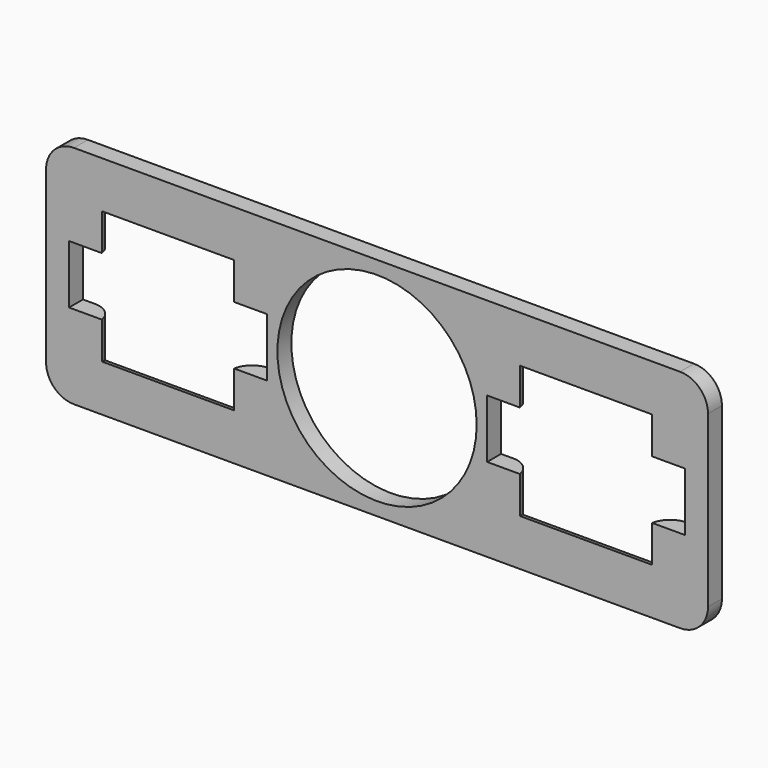
from build123d import *

# Parameters (mm, degrees)
F0_W          = 120.65
F0_H          = 41.148
F0_R          = 18.161
F1_DEPTH      = 3.175
F2_T1_DEPTH   = 24.13
F2_T3_DEPTH   = 16.1227766557
F2_T5_DEPTH   = 24.13
F2_T7_DEPTH   = 16.1227766557
F2_T13_DEPTH  = 16.1227766557
F2_T18_DEPTH  = 33.5217766557
F2_T25_DEPTH  = 33.5217766557
F2_T29_DEPTH  = 16.1227766557
F2_T37_DEPTH  = 33.5217766557
F2_T41_DEPTH  = 16.1227766557
F2_T49_DEPTH  = 16.1227766557
F2_T54_DEPTH  = 33.5217766557
F2_T61_DEPTH  = 33.5217766557
F2_T65_DEPTH  = 16.1227766557
F2_T73_DEPTH  = 16.1227766557
F2_T78_DEPTH  = 33.5217766557
F2_T85_DEPTH  = 33.5217766557
F2_T89_DEPTH  = 16.1227766557
F2_T97_DEPTH  = 16.1227766557
F2_T102_DEPTH = 33.5217766557
F3_R          = 5.08


# Not quite as in the source:
# - a fillet or chamfer that OpenCascade refuses, or shapes differently, is made with other operations: its cross-section is extruded or revolved along the edge and cut away or added
# - a feature names something its author has since deleted; it is built from what else it names


with BuildPart() as f1:
    # F0 (on Front) → F1 (new body)
    with BuildSketch(Plane.XZ):
        Rectangle(F0_W, F0_H)
        Polygon((-26.035, 5.334), (-20.066, 5.334), (-20.066, -5.334), (-26.035, -5.334), (-26.035, -12.065), (-50.165, -12.065), (-50.165, -5.334), (-56.134, -5.334), (-56.134, 5.334), (-50.165, 5.334), (-50.165, 12.065), (-26.035, 12.065), align=None, mode=Mode.SUBTRACT)
        Circle(F0_R, mode=Mode.SUBTRACT)
        Polygon((50.165, 5.334), (56.134, 5.334), (56.134, -5.334), (50.165, -5.334), (50.165, -12.065), (26.035, -12.065), (26.035, -5.334), (20.066, -5.334), (20.066, 5.334), (26.035, 5.334), (26.035, 12.065), (50.165, 12.065), align=None, mode=Mode.SUBTRACT)
    extrude(amount=F1_DEPTH)

    # F2: fillet of radius 3.81 on 12 edges, made by hand

    # F2_s2 → F2_t1 (cut)
    with BuildSketch(Plane.YZ.offset(26.035)):
        with BuildLine():
            ThreePointArc((-3.175, 12.065), (-0.9000644337, 13.3623662374), (0, 15.8217106623))
            Line((0, 15.8217106623), (0, 12.065))
            Line((0, 12.065), (-3.175, 12.065))
        make_face()
        with BuildLine():
            ThreePointArc((-3.175, -12.065), (-0.9000644337, -13.3623662374), (0, -15.8217106623))
            Line((0, -15.8217106623), (0, -12.065))
            Line((0, -12.065), (-3.175, -12.065))
        make_face()
    extrude(amount=F2_T1_DEPTH, mode=Mode.SUBTRACT)

    # F2_s4 → F2_t3 (cut)
    with BuildSketch(Plane.XY.offset(-4.0577766557)):
        with BuildLine():
            ThreePointArc((26.035, -3.175), (24.7376337626, -0.9000644337), (22.2782893377, 0))
            Line((22.2782893377, 0), (26.035, 0))
            Line((26.035, 0), (26.035, -3.175))
        make_face()
        with BuildLine():
            ThreePointArc((50.165, -3.175), (51.4623662374, -0.9000644337), (53.9217106623, 0))
            Line((53.9217106623, 0), (50.165, 0))
            Line((50.165, 0), (50.165, -3.175))
        make_face()
        with BuildLine():
            ThreePointArc((-26.035, -3.175), (-24.7376337626, -0.9000644337), (-22.2782893377, 0))
            Line((-22.2782893377, 0), (-26.035, 0))
            Line((-26.035, 0), (-26.035, -3.175))
        make_face()
        with BuildLine():
            ThreePointArc((-50.165, -3.175), (-51.4623662374, -0.9000644337), (-53.9217106623, 0))
            Line((-53.9217106623, 0), (-50.165, 0))
            Line((-50.165, 0), (-50.165, -3.175))
        make_face()
    extrude(amount=F2_T3_DEPTH, mode=Mode.SUBTRACT)

    # F2_s6 → F2_t5 (cut)
    with BuildSketch(Plane.YZ.offset(-50.165)):
        with BuildLine():
            ThreePointArc((-3.175, 12.065), (-0.9000644337, 13.3623662374), (0, 15.8217106623))
            Line((0, 15.8217106623), (0, 12.065))
            Line((0, 12.065), (-3.175, 12.065))
        make_face()
        with BuildLine():
            ThreePointArc((-3.175, -12.065), (-0.9000644337, -13.3623662374), (0, -15.8217106623))
            Line((0, -15.8217106623), (0, -12.065))
            Line((0, -12.065), (-3.175, -12.065))
        make_face()
    extrude(amount=F2_T5_DEPTH, mode=Mode.SUBTRACT)

    # F2_s8 → F2_t7 (cut)
    with BuildSketch(Plane.XY.offset(-12.065)):
        with BuildLine():
            ThreePointArc((-50.165, -3.175), (-51.4623662374, -0.9000644337), (-53.9217106623, 0))
            Line((-53.9217106623, 0), (-50.165, 0))
            Line((-50.165, 0), (-50.165, -3.175))
        make_face()
        with BuildLine():
            ThreePointArc((-26.035, -3.175), (-24.7376337626, -0.9000644337), (-22.2782893377, 0))
            Line((-22.2782893377, 0), (-26.035, 0))
            Line((-26.035, 0), (-26.035, -3.175))
        make_face()
        with BuildLine():
            ThreePointArc((26.035, -3.175), (24.7376337626, -0.9000644337), (22.2782893377, 0))
            Line((22.2782893377, 0), (26.035, 0))
            Line((26.035, 0), (26.035, -3.175))
        make_face()
        with BuildLine():
            ThreePointArc((50.165, -3.175), (51.4623662374, -0.9000644337), (53.9217106623, 0))
            Line((53.9217106623, 0), (50.165, 0))
            Line((50.165, 0), (50.165, -3.175))
        make_face()
    extrude(amount=F2_T7_DEPTH, mode=Mode.SUBTRACT)


with BuildPart() as f2_tool11:
    # F2_s12 → F2_t13 (new body)
    with BuildSketch(Plane.XY.offset(5.334)):
        with BuildLine():
            ThreePointArc((26.035, -3.175), (24.7376337626, -0.9000644337), (22.2782893377, 0))
            Line((22.2782893377, 0), (26.035, 0))
            Line((26.035, 0), (26.035, -3.175))
        make_face()
    extrude(amount=F2_T13_DEPTH)

    split(bisect_by=Plane.XY.offset(20.574), keep=Keep.BOTTOM)

    split(bisect_by=Plane.XY.offset(12.065), keep=Keep.TOP)


with BuildPart() as f2_tool16:
    # F2_s17 → F2_t18 (new body)
    with BuildSketch(Plane.YZ.offset(16.6432233443)):
        with BuildLine():
            ThreePointArc((-3.175, 12.065), (-0.9000644337, 13.3623662374), (0, 15.8217106623))
            Line((0, 15.8217106623), (0, 12.065))
            Line((0, 12.065), (-3.175, 12.065))
        make_face()
    extrude(amount=F2_T18_DEPTH)

    split(bisect_by=Plane.YZ.offset(26.035), keep=Keep.BOTTOM)


with BuildPart() as f2_tool11_1:
    add(f2_tool11.part)

    # F2_t20: intersect F2_tool16
    add(f2_tool16.part, mode=Mode.INTERSECT)


with BuildPart() as f1_1:
    add(f1.part)

    # F2_t9: cut F2_tool11
    add(f2_tool11_1.part, mode=Mode.SUBTRACT)


with BuildPart() as f2_tool23:
    # F2_s24 → F2_t25 (new body)
    with BuildSketch(Plane.YZ.offset(26.035)):
        with BuildLine():
            ThreePointArc((-3.175, 12.065), (-0.9000644337, 13.3623662374), (0, 15.8217106623))
            Line((0, 15.8217106623), (0, 12.065))
            Line((0, 12.065), (-3.175, 12.065))
        make_face()
    extrude(amount=F2_T25_DEPTH)

    split(bisect_by=Plane.YZ.offset(50.165), keep=Keep.TOP)


with BuildPart() as f2_tool27:
    # F2_s28 → F2_t29 (new body)
    with BuildSketch(Plane.XY.offset(21.4567766557)):
        with BuildLine():
            ThreePointArc((50.165, -3.175), (51.4623662374, -0.9000644337), (53.9217106623, 0))
            Line((53.9217106623, 0), (50.165, 0))
            Line((50.165, 0), (50.165, -3.175))
        make_face()
    extrude(amount=-F2_T29_DEPTH)

    split(bisect_by=Plane.XY.offset(20.574), keep=Keep.BOTTOM)

    split(bisect_by=Plane.XY.offset(12.065), keep=Keep.TOP)


with BuildPart() as f2_tool23_1:
    add(f2_tool23.part)

    # F2_t32: intersect F2_tool27
    add(f2_tool27.part, mode=Mode.INTERSECT)


with BuildPart() as f1_2:
    add(f1_1.part)

    # F2_t21: cut F2_tool23
    add(f2_tool23_1.part, mode=Mode.SUBTRACT)


with BuildPart() as f2_tool35:
    # F2_s36 → F2_t37 (new body)
    with BuildSketch(Plane.YZ.offset(-50.165)):
        with BuildLine():
            ThreePointArc((-3.175, 12.065), (-0.9000644337, 13.3623662374), (0, 15.8217106623))
            Line((0, 15.8217106623), (0, 12.065))
            Line((0, 12.065), (-3.175, 12.065))
        make_face()
    extrude(amount=F2_T37_DEPTH)

    split(bisect_by=Plane.YZ.offset(-26.035), keep=Keep.TOP)


with BuildPart() as f2_tool39:
    # F2_s40 → F2_t41 (new body)
    with BuildSketch(Plane.XY.offset(21.4567766557)):
        with BuildLine():
            ThreePointArc((-26.035, -3.175), (-24.7376337626, -0.9000644337), (-22.2782893377, 0))
            Line((-22.2782893377, 0), (-26.035, 0))
            Line((-26.035, 0), (-26.035, -3.175))
        make_face()
    extrude(amount=-F2_T41_DEPTH)

    split(bisect_by=Plane.XY.offset(20.574), keep=Keep.BOTTOM)

    split(bisect_by=Plane.XY.offset(12.065), keep=Keep.TOP)


with BuildPart() as f2_tool35_1:
    add(f2_tool35.part)

    # F2_t44: intersect F2_tool39
    add(f2_tool39.part, mode=Mode.INTERSECT)


with BuildPart() as f1_3:
    add(f1_2.part)

    # F2_t33: cut F2_tool35
    add(f2_tool35_1.part, mode=Mode.SUBTRACT)


with BuildPart() as f2_tool47:
    # F2_s48 → F2_t49 (new body)
    with BuildSketch(Plane.XY.offset(5.334)):
        with BuildLine():
            ThreePointArc((-50.165, -3.175), (-51.4623662374, -0.9000644337), (-53.9217106623, 0))
            Line((-53.9217106623, 0), (-50.165, 0))
            Line((-50.165, 0), (-50.165, -3.175))
        make_face()
    extrude(amount=F2_T49_DEPTH)

    split(bisect_by=Plane.XY.offset(20.574), keep=Keep.BOTTOM)

    split(bisect_by=Plane.XY.offset(12.065), keep=Keep.TOP)


with BuildPart() as f2_tool52:
    # F2_s53 → F2_t54 (new body)
    with BuildSketch(Plane.YZ.offset(-59.5567766557)):
        with BuildLine():
            ThreePointArc((-3.175, 12.065), (-0.9000644337, 13.3623662374), (0, 15.8217106623))
            Line((0, 15.8217106623), (0, 12.065))
            Line((0, 12.065), (-3.175, 12.065))
        make_face()
    extrude(amount=F2_T54_DEPTH)

    split(bisect_by=Plane.YZ.offset(-50.165), keep=Keep.BOTTOM)


with BuildPart() as f2_tool47_1:
    add(f2_tool47.part)

    # F2_t56: intersect F2_tool52
    add(f2_tool52.part, mode=Mode.INTERSECT)


with BuildPart() as f1_4:
    add(f1_3.part)

    # F2_t45: cut F2_tool47
    add(f2_tool47_1.part, mode=Mode.SUBTRACT)


with BuildPart() as f2_tool59:
    # F2_s60 → F2_t61 (new body)
    with BuildSketch(Plane.YZ.offset(-26.035)):
        with BuildLine():
            ThreePointArc((-3.175, -12.065), (-0.9000644337, -13.3623662374), (0, -15.8217106623))
            Line((0, -15.8217106623), (0, -12.065))
            Line((0, -12.065), (-3.175, -12.065))
        make_face()
    extrude(amount=-F2_T61_DEPTH)

    split(bisect_by=Plane.YZ.offset(-50.165), keep=Keep.BOTTOM)


with BuildPart() as f2_tool63:
    # F2_s64 → F2_t65 (new body)
    with BuildSketch(Plane.XY.offset(-21.4567766557)):
        with BuildLine():
            ThreePointArc((-50.165, -3.175), (-51.4623662374, -0.9000644337), (-53.9217106623, 0))
            Line((-53.9217106623, 0), (-50.165, 0))
            Line((-50.165, 0), (-50.165, -3.175))
        make_face()
    extrude(amount=F2_T65_DEPTH)

    split(bisect_by=Plane.XY.offset(-20.574), keep=Keep.TOP)

    split(bisect_by=Plane.XY.offset(-12.065), keep=Keep.BOTTOM)


with BuildPart() as f2_tool59_1:
    add(f2_tool59.part)

    # F2_t68: intersect F2_tool63
    add(f2_tool63.part, mode=Mode.INTERSECT)


with BuildPart() as f1_5:
    add(f1_4.part)

    # F2_t57: cut F2_tool59
    add(f2_tool59_1.part, mode=Mode.SUBTRACT)


with BuildPart() as f2_tool71:
    # F2_s72 → F2_t73 (new body)
    with BuildSketch(Plane.XY.offset(-5.334)):
        with BuildLine():
            ThreePointArc((-26.035, -3.175), (-24.7376337626, -0.9000644337), (-22.2782893377, 0))
            Line((-22.2782893377, 0), (-26.035, 0))
            Line((-26.035, 0), (-26.035, -3.175))
        make_face()
    extrude(amount=-F2_T73_DEPTH)

    split(bisect_by=Plane.XY.offset(-20.574), keep=Keep.TOP)

    split(bisect_by=Plane.XY.offset(-12.065), keep=Keep.BOTTOM)


with BuildPart() as f2_tool76:
    # F2_s77 → F2_t78 (new body)
    with BuildSketch(Plane.YZ.offset(-16.6432233443)):
        with BuildLine():
            ThreePointArc((-3.175, -12.065), (-0.9000644337, -13.3623662374), (0, -15.8217106623))
            Line((0, -15.8217106623), (0, -12.065))
            Line((0, -12.065), (-3.175, -12.065))
        make_face()
    extrude(amount=-F2_T78_DEPTH)

    split(bisect_by=Plane.YZ.offset(-26.035), keep=Keep.TOP)


with BuildPart() as f2_tool71_1:
    add(f2_tool71.part)

    # F2_t80: intersect F2_tool76
    add(f2_tool76.part, mode=Mode.INTERSECT)


with BuildPart() as f1_6:
    add(f1_5.part)

    # F2_t69: cut F2_tool71
    add(f2_tool71_1.part, mode=Mode.SUBTRACT)


with BuildPart() as f2_tool83:
    # F2_s84 → F2_t85 (new body)
    with BuildSketch(Plane.YZ.offset(50.165)):
        with BuildLine():
            ThreePointArc((-3.175, -12.065), (-0.9000644337, -13.3623662374), (0, -15.8217106623))
            Line((0, -15.8217106623), (0, -12.065))
            Line((0, -12.065), (-3.175, -12.065))
        make_face()
    extrude(amount=-F2_T85_DEPTH)

    split(bisect_by=Plane.YZ.offset(26.035), keep=Keep.BOTTOM)


with BuildPart() as f2_tool87:
    # F2_s88 → F2_t89 (new body)
    with BuildSketch(Plane.XY.offset(-21.4567766557)):
        with BuildLine():
            ThreePointArc((26.035, -3.175), (24.7376337626, -0.9000644337), (22.2782893377, 0))
            Line((22.2782893377, 0), (26.035, 0))
            Line((26.035, 0), (26.035, -3.175))
        make_face()
    extrude(amount=F2_T89_DEPTH)

    split(bisect_by=Plane.XY.offset(-20.574), keep=Keep.TOP)

    split(bisect_by=Plane.XY.offset(-12.065), keep=Keep.BOTTOM)


with BuildPart() as f2_tool83_1:
    add(f2_tool83.part)

    # F2_t92: intersect F2_tool87
    add(f2_tool87.part, mode=Mode.INTERSECT)


with BuildPart() as f1_7:
    add(f1_6.part)

    # F2_t81: cut F2_tool83
    add(f2_tool83_1.part, mode=Mode.SUBTRACT)


with BuildPart() as f2_tool95:
    # F2_s96 → F2_t97 (new body)
    with BuildSketch(Plane.XY.offset(-5.334)):
        with BuildLine():
            ThreePointArc((50.165, -3.175), (51.4623662374, -0.9000644337), (53.9217106623, 0))
            Line((53.9217106623, 0), (50.165, 0))
            Line((50.165, 0), (50.165, -3.175))
        make_face()
    extrude(amount=-F2_T97_DEPTH)

    split(bisect_by=Plane.XY.offset(-20.574), keep=Keep.TOP)

    split(bisect_by=Plane.XY.offset(-12.065), keep=Keep.BOTTOM)


with BuildPart() as f2_tool100:
    # F2_s101 → F2_t102 (new body)
    with BuildSketch(Plane.YZ.offset(59.5567766557)):
        with BuildLine():
            ThreePointArc((-3.175, -12.065), (-0.9000644337, -13.3623662374), (0, -15.8217106623))
            Line((0, -15.8217106623), (0, -12.065))
            Line((0, -12.065), (-3.175, -12.065))
        make_face()
    extrude(amount=-F2_T102_DEPTH)

    split(bisect_by=Plane.YZ.offset(50.165), keep=Keep.TOP)


with BuildPart() as f2_tool95_1:
    add(f2_tool95.part)

    # F2_t104: intersect F2_tool100
    add(f2_tool100.part, mode=Mode.INTERSECT)


with BuildPart() as f1_8:
    add(f1_7.part)

    # F2_t93: cut F2_tool95
    add(f2_tool95_1.part, mode=Mode.SUBTRACT)

    # F3
    f3_edges = [f1_8.edges().sort_by_distance(p)[0] for p in [
        (60.325, -1.5875, 20.574),
        (-60.325, -1.5875, 20.574),
        (-60.325, -1.5875, -20.574),
        (60.325, -1.5875, -20.574),
    ]]
    fillet(f3_edges, radius=F3_R)


solid = f1_8.part
